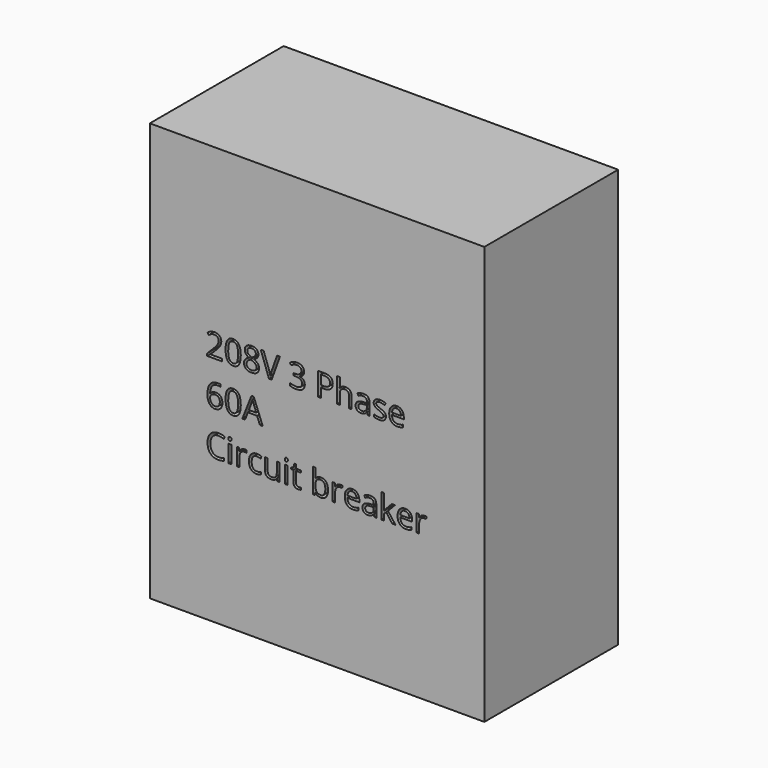
from build123d import *

# Parameters (mm, degrees)
F0_W         = 304.8
F0_H         = 381
F1_DEPTH     = 152.4
F2_TEXT_SIZE = 29.3178231661
F3_DEPTH     = 25.4


# Not quite as in the source:
# - Text() gives the source's letters only with a copy of the font that has no kerning and outlines rounded to 1/6400 em; it was checked with that copy


with BuildPart() as f1:
    # F0 (on Front) → F1 (new body)
    with BuildSketch(Plane.XZ):
        Rectangle(F0_W, F0_H)
    extrude(amount=F1_DEPTH)

    # F2 (on face) → F3 (cut)
    with BuildSketch(Plane.XZ.offset(152.4)):
        with Locations((-101.6, 20.9464588434)):
            Text('208V 3 Phase', F2_TEXT_SIZE, font='Open Sans', text_align=(TextAlign.LEFT, TextAlign.BOTTOM))
        with Locations((-101.6, -18.9257806625)):
            Text('60A', F2_TEXT_SIZE, font='Open Sans', text_align=(TextAlign.LEFT, TextAlign.BOTTOM))
        with Locations((-101.6, -58.7980201683)):
            Text('Circuit breaker', F2_TEXT_SIZE, font='Open Sans', text_align=(TextAlign.LEFT, TextAlign.BOTTOM))
    extrude(amount=-F3_DEPTH, mode=Mode.SUBTRACT)


solid = f1.part
